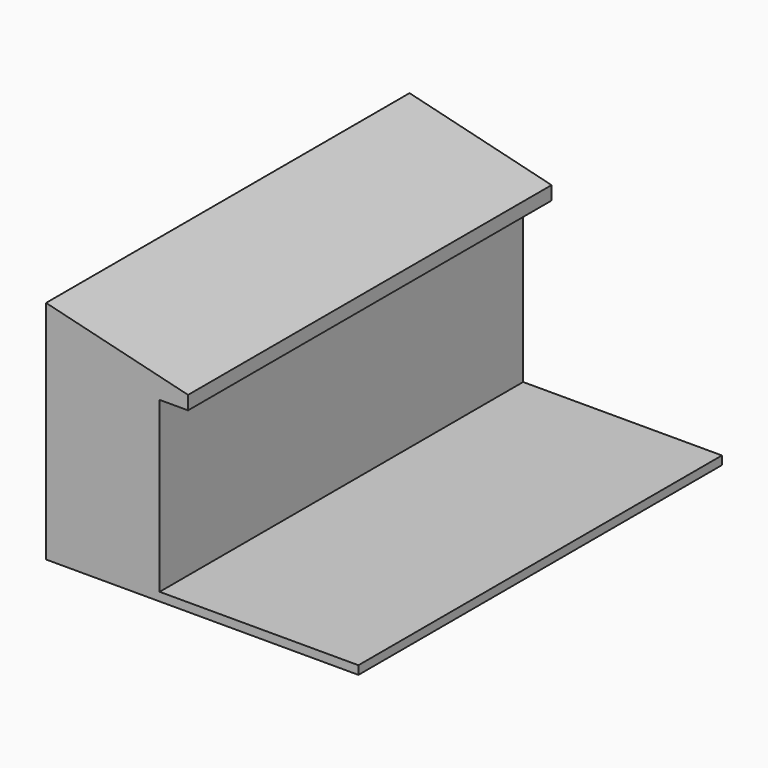
from build123d import *


# Not quite as in the source:
# - a feature names something its author has since deleted; it is built from what else it names


with BuildPart() as f2:
    # F2: sweep along a path in F1
    with BuildLine(Plane.YZ) as f2_path:
        Line((0, 0), (-8000, 0))
    # F0 (on Front) → F2 (sweep)
    with BuildSketch(Plane.XZ):
        Polygon((5500, 31.9677448273), (2000, 31.9677448273), (2000, 3006.9677448273), (2500, 3006.9677448273), (2500, 3246.9677448273), (0, 3860), (0, 0), (0, -118.0322551727), (5500, -118.0322551727), align=None)
    sweep(path=f2_path.line)


solid = f2.part
